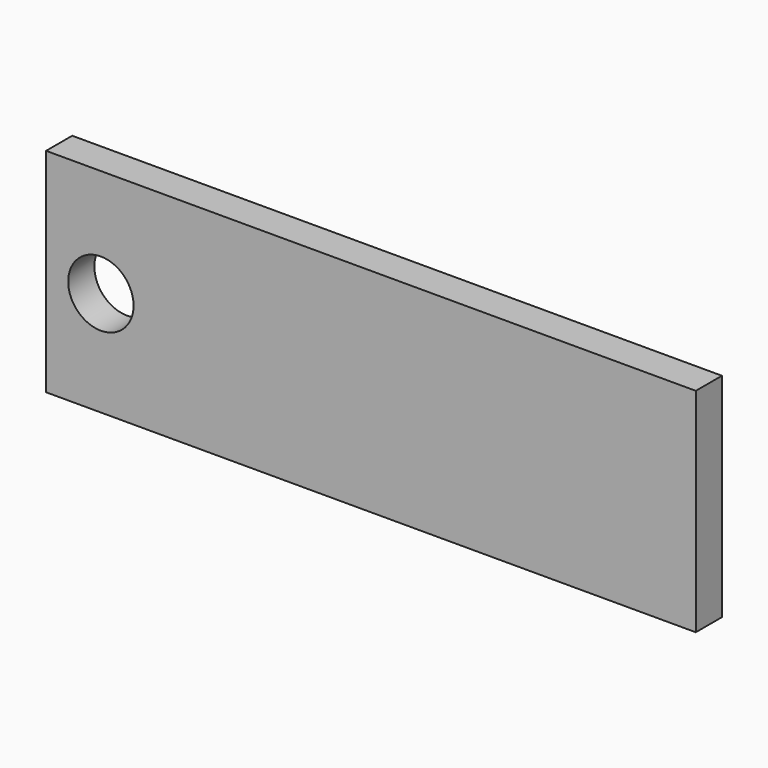
from build123d import *

# Parameters (mm, degrees)
F0_W           = 126.2744627893
F0_H           = 41.3146601059
F1_DEPTH       = 6.35
F2_W           = 102.6380173862
F2_H           = 32.7060690615
F3_DEPTH       = 2.54
F5_DEPTH       = 2.54
F4_TEXT_SIZE   = 34.9200207792
F6_DEPTH       = 2.54
F8_D           = 6.35
F8_CBORE_D     = 12.7
F8_CBORE_DEPTH = 6.35


# Not quite as in the source:
# - Text() gives the source's letters only with a copy of the font that has no kerning and outlines rounded to 1/6400 em; it was checked with that copy


with BuildPart() as f1:
    # F0 (on Front) → F1 (new body)
    with BuildSketch(Plane.XZ):
        with Locations((-12.9226837307, 17.6948390435)):
            Rectangle(F0_W, F0_H)
    extrude(amount=F1_DEPTH)

    # F2 (on Front) → F3 (cut)
    with BuildSketch(Plane.XZ):
        with Locations((-4.0988642722, 18.5772617115)):
            Rectangle(F2_W, F2_H)
    extrude(amount=F3_DEPTH, mode=Mode.SUBTRACT)

    # F8 (through all)
    with Locations(Plane(origin=(0, 0, 0), x_dir=(1, 0, 0), z_dir=(0, 1, 0))):
        with Locations((-65.4102861881, -17.386296764)):
            CounterBoreHole(F8_D / 2, F8_CBORE_D / 2, F8_CBORE_DEPTH)


with BuildPart() as f5:
    # F4 (on face) → F5 (new body)
    with BuildSketch(Plane(origin=(0, 0, 0), x_dir=(-1, 0, 0), z_dir=(0, 1, 0))):
        Polygon((38.3645756955, 6.8511082791), (44.3991917864, 6.8511082791), (35.9747367734, 19.4168595063), (43.7990039293, 31.7807293635), (38.1081317929, 31.7807293635), (32.8373911565, 22.8106490258), (27.4684379617, 31.7807293635), (21.635703241, 31.7807293635), (29.3781265981, 19.7060409284), (21.106446676, 6.8511082791), (26.7700375462, 6.8511082791), (32.5645784942, 16.2795138895), align=None)
    extrude(amount=F5_DEPTH)

    # F4 (on face) → F6 (join)
    with BuildSketch(Plane(origin=(0, 0, 0), x_dir=(-1, 0, 0), z_dir=(0, 1, 0))):
        with Locations((-42.2733910382, 6.8511082791)):
            Text('ALEX', F4_TEXT_SIZE, font='Open Sans', font_style=FontStyle.BOLD, text_align=(TextAlign.LEFT, TextAlign.BOTTOM))
    extrude(amount=F6_DEPTH)


solid = Compound([f1.part, f5.part])
